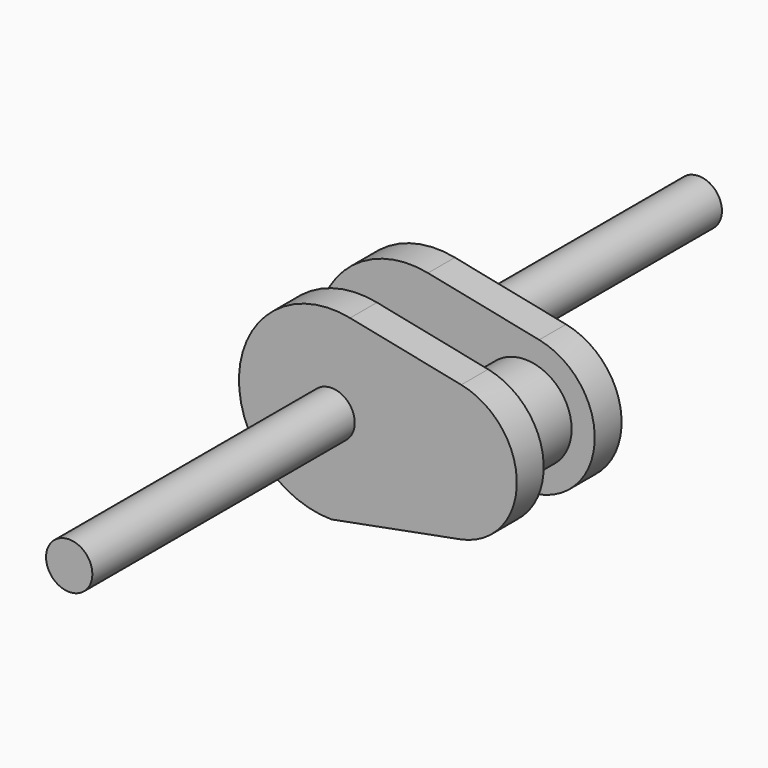
from build123d import *

# Parameters (mm, degrees)
F0_R     = 5.08
F0_R_2   = 10.16
F1_DEPTH = 7.366
F2_R     = 10.16
F3_DEPTH = 6.99897
F7_R     = 5.08
F8_DEPTH = 79.5782


# Not quite as in the source:
# - a length typed as a fraction of an inch, garbled in the dataset ("3 / 203.2 mm" for 3/8 in), is restored


with BuildPart() as f1:
    # F0 (on Front) → F1 (new body)
    with BuildSketch(Plane.XZ):
        with BuildLine():
            Line((28.448, 14.932089472), (4.064, 19.9094526293))
            ThreePointArc((4.064, 19.9094526293), (-20.2171026291, 2.0423421079), (0, -20.32))
            Line((0, -20.32), (7.4284633963, -18.9134960166))
            Line((7.4284633963, -18.9134960166), (28.2351667085, -14.9739583856))
            ThreePointArc((28.2351667085, -14.9739583856), (40.639614078, -0.1084562307), (28.448, 14.932089472))
        make_face()
        Circle(F0_R, mode=Mode.SUBTRACT)
        with Locations((25.4, 0)):
            Circle(F0_R_2, mode=Mode.SUBTRACT)
        with Locations((25.4, 0)):
            Circle(F0_R_2)
    extrude(amount=F1_DEPTH)

    # F2 (on face) → F3 (join)
    with BuildSketch(Plane.XZ.offset(7.366)):
        with Locations((25.4, 0)):
            Circle(F2_R)
    extrude(amount=F3_DEPTH)

    # F5: F1 across plane


with BuildPart() as f1_1:
    add(f1.part)
    add(f1.part.mirror(Plane(origin=(25.4, -14.36497, 0), x_dir=(1, 0, 0), z_dir=(0, -1, 0))))

    # F7 (on offset) → F8 (join)
    with BuildSketch(Plane.XZ.offset(21.10994)):
        Circle(F7_R)
    extrude(amount=F8_DEPTH)

    # F9: F1 across plane


with BuildPart() as f1_2:
    add(f1_1.part)
    add(f1_1.part.mirror(Plane(origin=(25.4, -14.36497, 0), x_dir=(1, 0, 0), z_dir=(0, -1, 0))))


solid = f1_2.part
